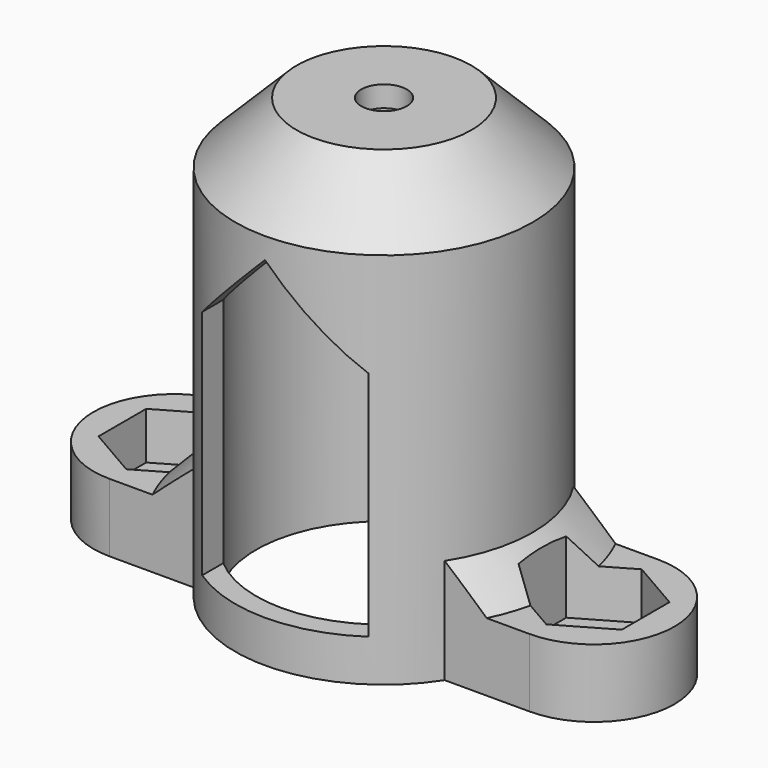
from build123d import *

# Parameters (mm, degrees)
F4_DEPTH       = 6
F9_DEPTH       = 4.251
F10_R          = 1.9
F11_DEPTH      = 1.2
F13_DEPTH      = 8.501
F13_DEPTH_BACK = 8.501
F15_R          = 1.3
F16_DEPTH      = 1.2


# Not quite as in the source:
# - a pattern or mirror of a feature is missing from the dataset's text; its kind, count and spacing are read off the source's solid


with BuildPart() as f2:
    # F1 (on Front) → F2 (revolve)
    with BuildSketch(Plane.XZ):
        Polygon((7.3, 37.5), (7.3, 16.4), (8.5, 16.4), (8.5, 37.9970562748), (4.9970562748, 41.5), (0, 41.5), (0, 40.3), (4.5, 40.3), align=None)
    revolve(axis=Axis((0, 0, 13.2), (0, 0, -1)))

    # F3 (on face) → F4 (join)
    with BuildSketch(Plane(origin=(0, 0, 16.4), x_dir=(1, 0, 0), z_dir=(0, 0, -1))):
        with BuildLine():
            Line((7.1477269114, -4.6), (12, -4.6))
            ThreePointArc((12, -4.6), (16.6, 0), (12, 4.6))
            Line((12, 4.6), (7.1477269114, 4.6))
            ThreePointArc((7.1477269114, 4.6), (8.5, 0), (7.1477269114, -4.6))
        make_face()
    f4 = extrude(amount=-F4_DEPTH)

    # F4_copies: F4 across plane
    add(f4.mirror(Plane(origin=(0, 0, 0), x_dir=(0, 0, -1), z_dir=(-1, 0, 0))))

    # F7 (on Front) → F8 (revolve, cut)
    with BuildSketch(Plane.XZ):
        Polygon((8.5, 22.4), (10.6, 20.3), (16.6, 20.3), (16.6, 22.4), align=None)
    revolve(axis=Axis((0, 0, 13.2), (0, 0, -1)), mode=Mode.SUBTRACT)

    # F6 (on offset) → F9 (cut, through all)
    with BuildSketch(Plane(origin=(0, 0, 17.6), x_dir=(1, 0, 0), z_dir=(0, 0, -1))):
        Polygon((12, -3.4063665882), (14.95, -1.7031832941), (14.95, 1.7031832941), (12, 3.4063665882), (9.05, 1.7031832941), (9.05, -1.7031832941), align=None)
    f9 = extrude(amount=-F9_DEPTH, mode=Mode.SUBTRACT)

    # F9_copies: F9 across plane
    add(f9.mirror(Plane(origin=(0, 0, 0), x_dir=(0, 0, -1), z_dir=(-1, 0, 0))), mode=Mode.SUBTRACT)

    # F10 (on face) → F11 (cut, through all)
    with BuildSketch(Plane(origin=(0, 0, 16.4), x_dir=(1, 0, 0), z_dir=(0, 0, -1))):
        with Locations((12, 0)):
            Circle(F10_R)
    f11 = extrude(amount=-F11_DEPTH, mode=Mode.SUBTRACT)

    # F11_copies: F11 across plane
    add(f11.mirror(Plane(origin=(0, 0, 0), x_dir=(0, 0, -1), z_dir=(-1, 0, 0))), mode=Mode.SUBTRACT)

    # F12 (on Front) → F13 (cut, two sides)
    with BuildSketch(Plane.XZ) as f13_sk:
        Polygon((-4.75, 32.0470562748), (-4.75, 18.8), (4.75, 18.8), (4.75, 32.0470562748), (0, 36.7970562748), align=None)
    extrude(amount=-F13_DEPTH, mode=Mode.SUBTRACT)
    extrude(f13_sk.sketch, amount=F13_DEPTH_BACK, mode=Mode.SUBTRACT)

    # F15 (on face) → F16 (cut, through all)
    with BuildSketch(Plane.XY.offset(41.5)):
        Circle(F15_R)
    extrude(amount=-F16_DEPTH, mode=Mode.SUBTRACT)


solid = f2.part
